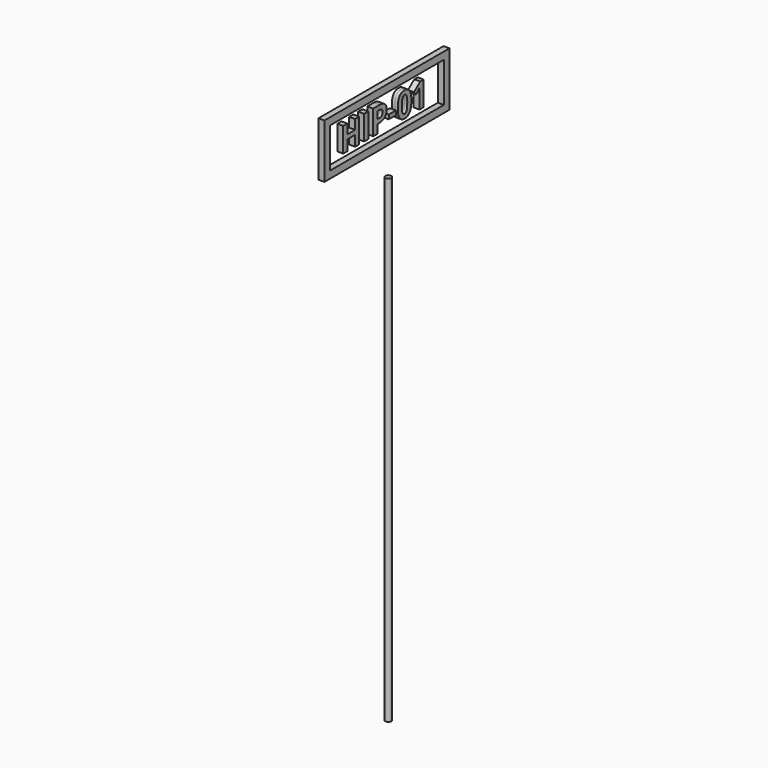
from build123d import *

# Parameters (mm, degrees)
F0_R         = 76.2
F1_DEPTH     = 12192
F3_W         = 3986.2990379333
F3_H         = 1379.5109987259
F3_W_2       = 3620.5389499664
F3_H_2       = 1013.750910759
F4_DEPTH     = 76.2
F2_TEXT_SIZE = 871.6113244494
F5_DEPTH     = 76.2


# Not quite as in the source:
# - Text() gives the source's letters only with a copy of the font that has no kerning and outlines rounded to 1/6400 em; it was checked with that copy


with BuildPart() as f1:
    # F0 (on Top) → F1 (new body)
    with BuildSketch(Plane.XY):
        Circle(F0_R)
    extrude(amount=-F1_DEPTH)


with BuildPart() as f4:
    # F3 (on Right) → F4 (new body, symmetric)
    with BuildSketch(Plane.YZ):
        with Locations((-137.122631073, 1469.0191149712)):
            Rectangle(F3_W, F3_H)
        with Locations((-137.122631073, 1469.0191149712)):
            Rectangle(F3_W_2, F3_H_2, mode=Mode.SUBTRACT)
    extrude(amount=F4_DEPTH, both=True)


with BuildPart() as f5:
    # F2 (on Right) → F5 (new body, symmetric)
    with BuildSketch(Plane.YZ):
        with Locations((-1609.4750165939, 1171.3307201862)):
            Text('HIP-01', F2_TEXT_SIZE, font='Open Sans', font_style=FontStyle.BOLD, text_align=(TextAlign.LEFT, TextAlign.BOTTOM))
    extrude(amount=F5_DEPTH, both=True)


solid = Compound([f1.part, f4.part, f5.part])
